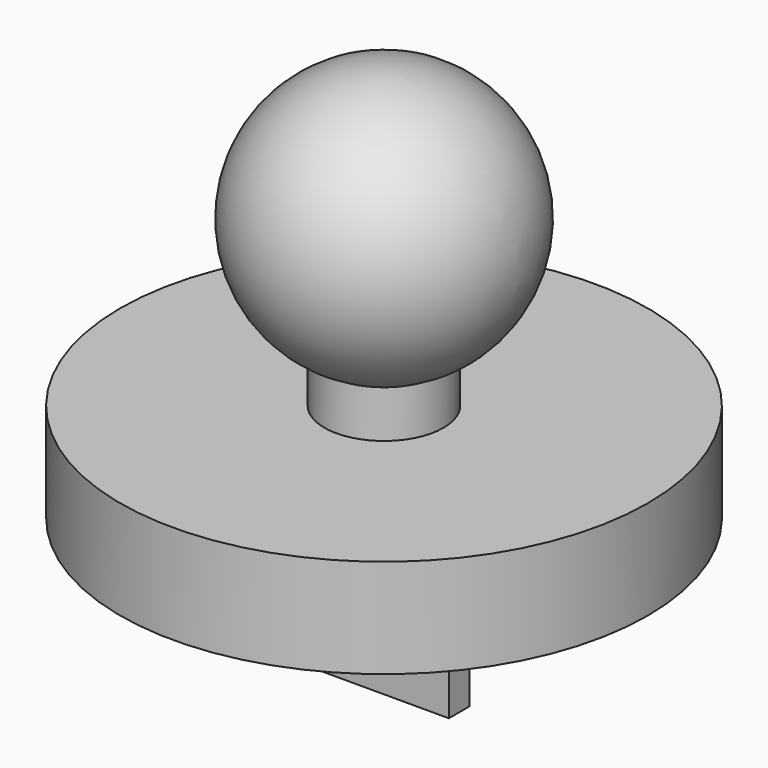
from build123d import *

# Parameters (mm, degrees)
F0_W           = 25.4
F0_H           = 12.7
F2_TEXT_SIZE   = 32.3711959128
F2_TEXT_SIZE_2 = 33.3374999981
F3_DEPTH       = 12.7
F4_R           = 25.4
F5_DEPTH       = 12.7


# Not quite as in the source:
# - Text() gives the source's letters only with a copy of the font that has no kerning and outlines rounded to 1/6400 em; it was checked with that copy


with BuildPart() as f1:
    # F0 (on Front) → F1 (revolve)
    with BuildSketch(Plane.XZ):
        with BuildLine():
            Line((0, 38.1), (0, 0))
            Line((0, 0), (25.4, 0))
            Line((25.4, 0), (25.4, 9.525))
            Line((25.4, 9.525), (5.7401240197, 9.525))
            Line((5.7401240197, 9.525), (5.7401240197, 14.0712323601))
            ThreePointArc((5.7401240197, 14.0712323601), (12.3524359749, 28.3508177658), (0, 38.1))
        make_face()
    revolve(axis=Axis((0, 0, -12.7), (0, 0, 1)))


with BuildPart() as f1b:
    # F0 (on Front) → F1, piece 2 (revolve)
    with BuildSketch(Plane.XZ):
        with Locations((12.7, -12.7)):
            Rectangle(F0_W, F0_H)
    revolve(axis=Axis((0, 0, -12.7), (0, 0, 1)))

    # F2 (on face) → F3 (join)
    with BuildSketch(Plane.XY.offset(-6.35)):
        with Locations((-18.3150156875, -12.1774123982)):
            Text('S', F2_TEXT_SIZE, font='Open Sans', text_align=(TextAlign.LEFT, TextAlign.BOTTOM))
        with Locations((0, -12.8731513396)):
            Text('L', F2_TEXT_SIZE_2, font='Open Sans', text_align=(TextAlign.LEFT, TextAlign.BOTTOM))
    extrude(amount=F3_DEPTH)

    # F4 (on face) → F5 (cut)
    with BuildSketch(Plane(origin=(0, 0, -19.05), x_dir=(1, 0, 0), z_dir=(0, 0, -1))):
        Circle(F4_R)
    extrude(amount=-F5_DEPTH, mode=Mode.SUBTRACT)


solid = Compound([f1.part, f1b.part])
